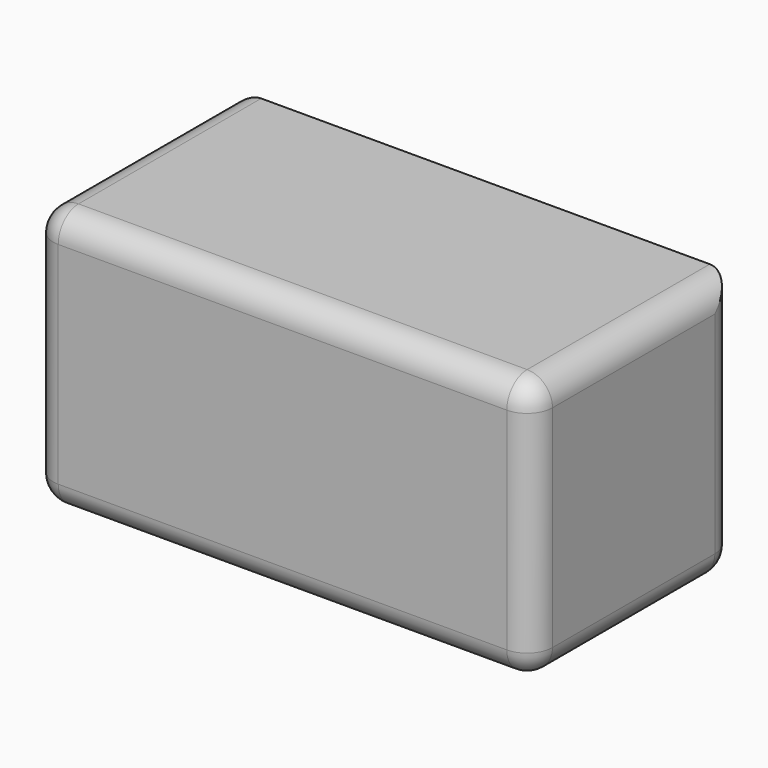
from build123d import *

# Parameters (mm, degrees)
F0_W         = 98.4050109982
F0_H         = 51.5961423516
F1_DEPTH     = 25
F2_R         = 5
F3_T1_DEPTH  = 76.5961423516
F3_T3_DEPTH  = 57.5
F3_S7_W      = 5
F3_S7_H      = 5
F3_T8_DEPTH  = 5
F3_S13_W     = 5
F3_S13_H     = 5
F3_T14_DEPTH = 5
F4_T1_DEPTH  = 40
F4_T3_DEPTH  = 88.4050109982
F4_S7_W      = 5
F4_S7_H      = 5
F4_T8_DEPTH  = 5
F4_S13_W     = 5
F4_S13_H     = 5
F4_T14_DEPTH = 5
F4_T18_ANGLE = 90


# Not quite as in the source:
# - a fillet or chamfer that OpenCascade refuses, or shapes differently, is made with other operations: its cross-section is extruded or revolved along the edge and cut away or added


with BuildPart() as f1:
    # F0 (on Front) → F1 (new body, symmetric)
    with BuildSketch(Plane.XZ):
        with Locations((-49.2025054991, 25.7980711758)):
            Rectangle(F0_W, F0_H)
    extrude(amount=F1_DEPTH, both=True)

    # F2
    f2_edges = [f1.edges().sort_by_distance(p)[0] for p in [
        (0, -25, 25.798071),
        (0, 0, 51.596142),
        (0, 25, 25.798071),
        (-49.202505, -25, 51.596142),
        (-49.202505, -25, 0),
        (-98.405011, -25, 25.798071),
    ]]
    fillet(f2_edges, radius=F2_R)

    # F3: fillet of radius 5 on 3 edges, made by hand

    # F3_s2 → F3_t1 (cut)
    with BuildSketch(Plane.XY.offset(-12.5)):
        with BuildLine():
            ThreePointArc((-93.4050109982, 25), (-96.9405449042, 23.5355339059), (-98.4050109982, 20))
            Line((-98.4050109982, 20), (-98.4050109982, 25))
            Line((-98.4050109982, 25), (-93.4050109982, 25))
        make_face()
    extrude(amount=F3_T1_DEPTH, mode=Mode.SUBTRACT)

    # F3_s4 → F3_t3 (cut)
    with BuildSketch(Plane.XZ.offset(-37.5)):
        with BuildLine():
            ThreePointArc((-98.4050109982, 46.5961423516), (-96.9405449042, 50.1316762576), (-93.4050109982, 51.5961423516))
            Line((-93.4050109982, 51.5961423516), (-98.4050109982, 51.5961423516))
            Line((-98.4050109982, 51.5961423516), (-98.4050109982, 46.5961423516))
        make_face()
        with BuildLine():
            ThreePointArc((-93.4050109982, 0), (-96.9405449042, 1.4644660941), (-98.4050109982, 5))
            Line((-98.4050109982, 5), (-98.4050109982, 0))
            Line((-98.4050109982, 0), (-93.4050109982, 0))
        make_face()
    extrude(amount=F3_T3_DEPTH, mode=Mode.SUBTRACT)


with BuildPart() as f3_tool6:
    # F3_s7 → F3_t8 (new body)
    with BuildSketch(Plane.XY.offset(5)):
        with Locations((-95.9050109982, -22.5)):
            Rectangle(F3_S7_W, F3_S7_H)
    extrude(amount=-F3_T8_DEPTH)

    # F3_s9 → F3_t10 (revolve, cut)
    with BuildSketch(Plane(origin=(-93.4050109982, -20, 5), x_dir=(0.7071067812, 0.7071067812, 0), z_dir=(-0.7071067812, 0.7071067812, 0))):
        with BuildLine():
            ThreePointArc((0, -5), (5, 0), (0, 5))
            Line((0, 5), (0, -5))
        make_face()
    revolve(axis=Axis((-93.4050109982, -20, 5), (0, 0, -1)), mode=Mode.SUBTRACT)


with BuildPart() as f1_1:
    add(f1.part)

    # F3_t5: cut F3_tool6
    add(f3_tool6.part, mode=Mode.SUBTRACT)


with BuildPart() as f3_tool12:
    # F3_s13 → F3_t14 (new body)
    with BuildSketch(Plane.YZ.offset(-93.4050109982)):
        with Locations((-22.5, 49.0961423516)):
            Rectangle(F3_S13_W, F3_S13_H)
    extrude(amount=-F3_T14_DEPTH)

    # F3_s15 → F3_t16 (revolve, cut)
    with BuildSketch(Plane(origin=(-93.4050109982, -20, 46.5961423516), x_dir=(0, 0.7071067812, -0.7071067812), z_dir=(0, 0.7071067812, 0.7071067812))):
        with BuildLine():
            ThreePointArc((0, -5), (5, 0), (0, 5))
            Line((0, 5), (0, -5))
        make_face()
    revolve(axis=Axis((-93.4050109982, -20, 46.5961423516), (-1, 0, 0)), mode=Mode.SUBTRACT)


with BuildPart() as f1_2:
    add(f1_1.part)

    # F3_t11: cut F3_tool12
    add(f3_tool12.part, mode=Mode.SUBTRACT)

    # F4: fillet of radius 5 on 1 edges, made by hand

    # F4_s2 → F4_t1 (cut)
    with BuildSketch(Plane.XZ.offset(-20)):
        with BuildLine():
            ThreePointArc((-5, 0), (-1.4644660941, 1.4644660941), (0, 5))
            Line((0, 5), (0, 0))
            Line((0, 0), (-5, 0))
        make_face()
    extrude(amount=F4_T1_DEPTH, mode=Mode.SUBTRACT)

    # F4_s4 → F4_t3 (cut)
    with BuildSketch(Plane.YZ.offset(-93.4050109982)):
        with BuildLine():
            ThreePointArc((20, 0), (23.5355339059, 1.4644660941), (25, 5))
            Line((25, 5), (25, 0))
            Line((25, 0), (20, 0))
        make_face()
    extrude(amount=F4_T3_DEPTH, mode=Mode.SUBTRACT)


with BuildPart() as f4_tool6:
    # F4_s7 → F4_t8 (new body)
    with BuildSketch(Plane.XY.offset(5)):
        with Locations((-2.5, -22.5)):
            Rectangle(F4_S7_W, F4_S7_H)
    extrude(amount=-F4_T8_DEPTH)

    # F4_s9 → F4_t10 (revolve, cut)
    with BuildSketch(Plane(origin=(-5, -20, 5), x_dir=(-0.7071067812, 0.7071067812, 0), z_dir=(-0.7071067812, -0.7071067812, 0))):
        with BuildLine():
            ThreePointArc((0, -5), (5, 0), (0, 5))
            Line((0, 5), (0, -5))
        make_face()
    revolve(axis=Axis((-5, -20, 5), (0, 0, -1)), mode=Mode.SUBTRACT)


with BuildPart() as f1_3:
    add(f1_2.part)

    # F4_t5: cut F4_tool6
    add(f4_tool6.part, mode=Mode.SUBTRACT)


with BuildPart() as f4_tool12:
    # F4_s13 → F4_t14 (new body)
    with BuildSketch(Plane.XY.offset(5)):
        with Locations((-95.9050109982, 22.5)):
            Rectangle(F4_S13_W, F4_S13_H)
    extrude(amount=-F4_T14_DEPTH)

    # F4_s15 → F4_t16 (revolve, cut)
    with BuildSketch(Plane(origin=(-93.4050109982, 20, 5), x_dir=(0.7071067812, -0.7071067812, 0), z_dir=(0.7071067812, 0.7071067812, 0))):
        with BuildLine():
            ThreePointArc((0, -5), (5, 0), (0, 5))
            Line((0, 5), (0, -5))
        make_face()
    revolve(axis=Axis((-93.4050109982, 20, 5), (0, 0, -1)), mode=Mode.SUBTRACT)


with BuildPart() as f1_4:
    add(f1_3.part)

    # F4_t11: cut F4_tool12
    add(f4_tool12.part, mode=Mode.SUBTRACT)

    # F4_s17 → F4_t18 (revolve, cut)
    with BuildSketch(Plane.XZ.offset(-20)):
        with BuildLine():
            ThreePointArc((-5, 0), (-1.4644660941, 1.4644660941), (0, 5))
            Line((0, 5), (0, 0))
            Line((0, 0), (-5, 0))
        make_face()
    revolve(axis=Axis((-5, 20, 0), (0, 0, 1)), revolution_arc=F4_T18_ANGLE, mode=Mode.SUBTRACT)


solid = f1_4.part
